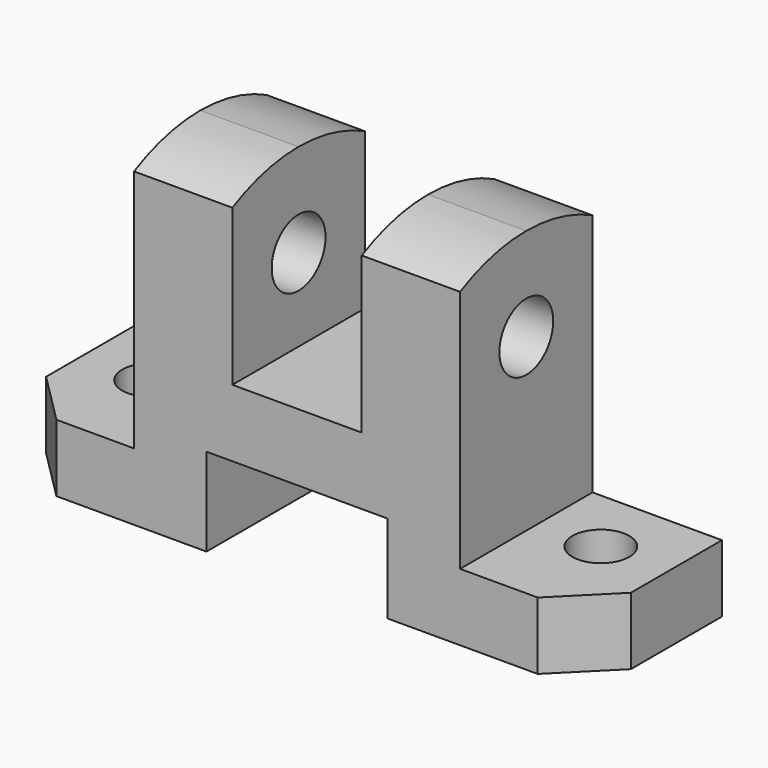
from build123d import *

# Parameters (mm, degrees)
F1_DEPTH      = 16
F3_DEPTH      = 56.501
F3_DEPTH_BACK = 56.501
F4_SIZE       = 10
F5_SIZE       = 10
F6_R          = 5.5
F7_DEPTH      = 64.001
F8_R          = 6.5
F9_DEPTH      = 88.001


with BuildPart() as f1:
    # F0 (on Front) → F1 (new body, symmetric)
    with BuildSketch(Plane.XZ):
        Polygon((-56.5, 13), (-56.5, 0), (-17.5, 0), (-17.5, 17), (17.5, 17), (17.5, 0), (56.5, 0), (56.5, 13), (31.5, 13), (31.5, 64), (12.5, 64), (12.5, 30), (-12.5, 30), (-12.5, 64), (-31.5, 64), (-31.5, 13), align=None)
    extrude(amount=F1_DEPTH, both=True)

    # F2 (on Right) → F3 (cut, two sides)
    with BuildSketch(Plane.YZ) as f3_sk:
        with BuildLine():
            Line((16, 64), (0, 64))
            ThreePointArc((0, 64), (8.230833216, 63.0184271325), (16, 60.1287648325))
            Line((16, 60.1287648325), (16, 64))
        make_face()
        with BuildLine():
            Line((0, 64), (-16, 64))
            Line((-16, 64), (-16, 60.1287648325))
            ThreePointArc((-16, 60.1287648325), (-8.2308332161, 63.0184271325), (0, 64))
        make_face()
    extrude(amount=-F3_DEPTH, mode=Mode.SUBTRACT)
    extrude(f3_sk.sketch, amount=F3_DEPTH_BACK, mode=Mode.SUBTRACT)

    # F4
    f4_edges = [f1.edges().sort_by_distance(p)[0] for p in [
        (56.5, -16, 6.5),
    ]]
    chamfer(f4_edges, length=F4_SIZE)

    # F5
    f5_edges = [f1.edges().sort_by_distance(p)[0] for p in [
        (-56.5, -16, 6.5),
    ]]
    chamfer(f5_edges, length=F5_SIZE)

    # F6 (on Top) → F7 (cut, through all)
    with BuildSketch(Plane.XY):
        with Locations((-43.5, 3)):
            Circle(F6_R)
        with Locations((43.5, 3)):
            Circle(F6_R)
    extrude(amount=F7_DEPTH, mode=Mode.SUBTRACT)

    # F8 (on face) → F9 (cut, through all)
    with BuildSketch(Plane.YZ.offset(31.5)):
        with Locations((0, 46)):
            Circle(F8_R)
    extrude(amount=-F9_DEPTH, mode=Mode.SUBTRACT)


solid = f1.part
